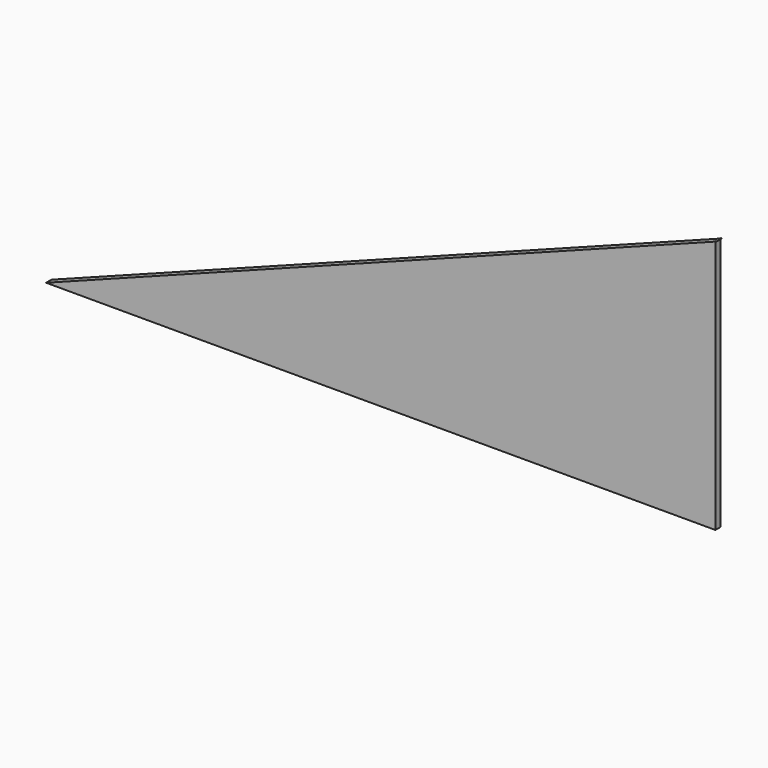
from build123d import *

# Parameters (mm, degrees)
F1_DEPTH = 0.5


# Not quite as in the source:
# - a feature names something its author has since deleted; it is built from what else it names


with BuildPart() as f1:
    # F0 (on Front) → F1 (new body)
    with BuildSketch(Plane.XZ):
        Polygon((0, 18.9663409947), (-50, 0), (0, 0), align=None)
    extrude(amount=F1_DEPTH)


with BuildPart() as f1b:
    # F0 (on Front) → F1, piece 2 (new body)
    with BuildSketch(Plane.XZ):
        Polygon((0, 19), (0, 18.9663409947), (0.0887335236, 19), align=None)
    extrude(amount=F1_DEPTH)


solid = Compound([f1.part, f1b.part])
